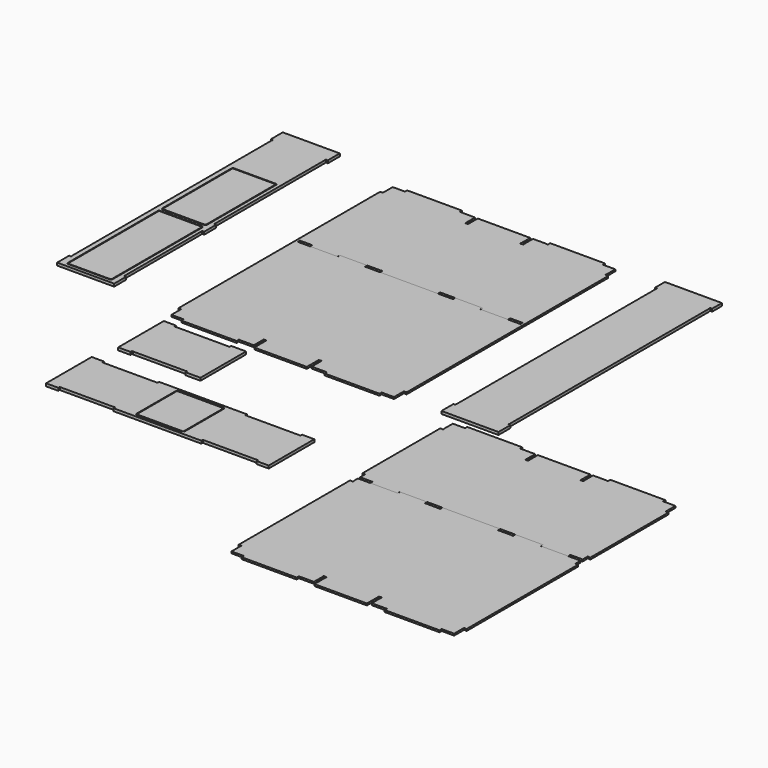
from build123d import *

# Parameters (mm, degrees)
F3_DEPTH  = 12
F5_DEPTH  = 18
F7_DEPTH  = 18
F9_DEPTH  = 18
F11_DEPTH = 12
F13_DEPTH = 12
F14_DEPTH = 18
F15_DEPTH = 12


with BuildPart() as f3:
    # F2 (on Top) → F3 (new body)
    with BuildSketch(Plane.XY):
        with BuildLine():
            Line((-993.5265209191, 1782.8284271247), (-1360.5265209191, 1782.8284271247))
            Line((-1360.5265209191, 1782.8284271247), (-1360.5265209191, 1770.8604506609))
            ThreePointArc((-1360.5265209191, 1770.8604506609), (-1359.5132677477, 1769.5012526055), (-1359.1540050798, 1767.8444388928))
            ThreePointArc((-1359.1540050798, 1767.8444388928), (-1359.5132677477, 1766.1876251801), (-1360.5265209191, 1764.8284271247))
            ThreePointArc((-1360.5265209191, 1764.8284271247), (-1363.1540050798, 1763.8444388928), (-1365.7814892405, 1764.8284271247))
            Line((-1365.7814892405, 1764.8284271247), (-1442.5265209191, 1764.8284271247))
            Line((-1442.5265209191, 1764.8284271247), (-1442.5265209191, 1688.4852813742))
            ThreePointArc((-1442.5265209191, 1688.4852813742), (-1441.6594299138, 1687.187587979), (-1441.3549480438, 1685.6568542495))
            ThreePointArc((-1441.3549480438, 1685.6568542495), (-1441.6594299138, 1684.12612052), (-1442.5265209191, 1682.8284271247))
            ThreePointArc((-1442.5265209191, 1682.8284271247), (-1445.3549480438, 1681.6568542495), (-1448.1833751686, 1682.8284271247))
            Line((-1448.1833751686, 1682.8284271247), (-1460.5265209191, 1682.8284271247))
            Line((-1460.5265209191, 1682.8284271247), (-1460.5265209191, 993.8284271247))
            Line((-1460.5265209191, 993.8284271247), (-1460.5265209191, 991.8284271247))
            Line((-1460.5265209191, 991.8284271247), (-1442.5265209191, 991.8284271247))
            Line((-1442.5265209191, 991.8284271247), (-1366.1833751686, 991.8284271247))
            ThreePointArc((-1366.1833751686, 991.8284271247), (-1363.3549480438, 993), (-1360.5265209191, 991.8284271247))
            ThreePointArc((-1360.5265209191, 991.8284271247), (-1359.6594299138, 990.5307337295), (-1359.3549480438, 989))
            ThreePointArc((-1359.3549480438, 989), (-1359.6594299138, 987.4692662705), (-1360.5265209191, 986.1715728753))
            Line((-1360.5265209191, 986.1715728753), (-1360.5265209191, 973.8284271247))
            Line((-1360.5265209191, 973.8284271247), (-1182.6833751686, 973.8284271247))
            Line((-1182.6833751686, 973.8284271247), (-1177.0265209191, 973.8284271247))
            Line((-1177.0265209191, 973.8284271247), (-1177.0265209191, 979.4852813742))
            Line((-1177.0265209191, 979.4852813742), (-1177.0265209191, 986.1715728753))
            ThreePointArc((-1177.0265209191, 986.1715728753), (-1178.1980937943, 989), (-1177.0265209191, 991.8284271247))
            ThreePointArc((-1177.0265209191, 991.8284271247), (-1174.1980937943, 993), (-1171.3696666696, 991.8284271247))
            Line((-1171.3696666696, 991.8284271247), (-993.5265209191, 991.8284271247))
            Line((-993.5265209191, 991.8284271247), (-899.1833751686, 991.8284271247))
            ThreePointArc((-899.1833751686, 991.8284271247), (-896.3549480438, 993), (-893.5265209191, 991.8284271247))
            ThreePointArc((-893.5265209191, 991.8284271247), (-892.6594299138, 990.5307337295), (-892.3549480438, 989))
            ThreePointArc((-892.3549480438, 989), (-892.6594299138, 987.4692662705), (-893.5265209191, 986.1715728753))
            Line((-893.5265209191, 986.1715728753), (-893.5265209191, 973.8284271247))
            Line((-893.5265209191, 973.8284271247), (-507.5265209191, 973.8284271247))
            Line((-507.5265209191, 973.8284271247), (-507.5265209191, 986.1715728753))
            ThreePointArc((-507.5265209191, 986.1715728753), (-508.6980937943, 989), (-507.5265209191, 991.8284271247))
            ThreePointArc((-507.5265209191, 991.8284271247), (-504.6980937943, 993), (-501.8696666696, 991.8284271247))
            Line((-501.8696666696, 991.8284271247), (-407.5265209191, 991.8284271247))
            Line((-407.5265209191, 991.8284271247), (-229.6833751686, 991.8284271247))
            ThreePointArc((-229.6833751686, 991.8284271247), (-226.8549480438, 993), (-224.0265209191, 991.8284271247))
            ThreePointArc((-224.0265209191, 991.8284271247), (-222.8549480438, 989), (-224.0265209191, 986.1715728753))
            Line((-224.0265209191, 986.1715728753), (-224.0265209191, 979.4852813742))
            Line((-224.0265209191, 979.4852813742), (-224.0265209191, 973.8284271247))
            Line((-224.0265209191, 973.8284271247), (-218.3696666696, 973.8284271247))
            Line((-218.3696666696, 973.8284271247), (-40.5265209191, 973.8284271247))
            Line((-40.5265209191, 973.8284271247), (-40.5265209191, 986.1715728753))
            ThreePointArc((-40.5265209191, 986.1715728753), (-41.6980937943, 989), (-40.5265209191, 991.8284271247))
            ThreePointArc((-40.5265209191, 991.8284271247), (-37.6980937943, 993), (-34.8696666696, 991.8284271247))
            Line((-34.8696666696, 991.8284271247), (41.4734790809, 991.8284271247))
            Line((41.4734790809, 991.8284271247), (59.4734790809, 991.8284271247))
            Line((59.4734790809, 991.8284271247), (59.4734790809, 993.8284271247))
            Line((59.4734790809, 993.8284271247), (59.4734790809, 1682.8284271247))
            Line((59.4734790809, 1682.8284271247), (47.1303333304, 1682.8284271247))
            ThreePointArc((47.1303333304, 1682.8284271247), (44.3019062057, 1681.6568542495), (41.4734790809, 1682.8284271247))
            ThreePointArc((41.4734790809, 1682.8284271247), (40.3019062057, 1685.6568542495), (41.4734790809, 1688.4852813742))
            Line((41.4734790809, 1688.4852813742), (41.4734790809, 1764.8284271247))
            Line((41.4734790809, 1764.8284271247), (-35.2715525977, 1764.8284271247))
            ThreePointArc((-35.2715525977, 1764.8284271247), (-37.8990367584, 1763.8444388928), (-40.5265209191, 1764.8284271247))
            ThreePointArc((-40.5265209191, 1764.8284271247), (-41.8990367584, 1767.8444388928), (-40.5265209191, 1770.8604506609))
            Line((-40.5265209191, 1770.8604506609), (-40.5265209191, 1782.8284271247))
            Line((-40.5265209191, 1782.8284271247), (-407.5265209191, 1782.8284271247))
            Line((-407.5265209191, 1782.8284271247), (-407.5265209191, 1770.4852813742))
            ThreePointArc((-407.5265209191, 1770.4852813742), (-406.6594299138, 1769.187587979), (-406.3549480438, 1767.6568542495))
            ThreePointArc((-406.3549480438, 1767.6568542495), (-406.6594299138, 1766.12612052), (-407.5265209191, 1764.8284271247))
            ThreePointArc((-407.5265209191, 1764.8284271247), (-410.3549480438, 1763.6568542495), (-413.1833751686, 1764.8284271247))
            Line((-413.1833751686, 1764.8284271247), (-507.5265209191, 1764.8284271247))
            Line((-507.5265209191, 1764.8284271247), (-507.5265209191, 1688.4852813742))
            ThreePointArc((-507.5265209191, 1688.4852813742), (-506.6594299138, 1687.187587979), (-506.3549480438, 1685.6568542495))
            ThreePointArc((-506.3549480438, 1685.6568542495), (-506.6594299138, 1684.12612052), (-507.5265209191, 1682.8284271247))
            ThreePointArc((-507.5265209191, 1682.8284271247), (-510.3549480438, 1681.6568542495), (-513.1833751686, 1682.8284271247))
            Line((-513.1833751686, 1682.8284271247), (-519.8696666696, 1682.8284271247))
            ThreePointArc((-519.8696666696, 1682.8284271247), (-522.6980937943, 1681.6568542495), (-525.5265209191, 1682.8284271247))
            ThreePointArc((-525.5265209191, 1682.8284271247), (-526.6980937943, 1685.6568542495), (-525.5265209191, 1688.4852813742))
            Line((-525.5265209191, 1688.4852813742), (-525.5265209191, 1764.8284271247))
            Line((-525.5265209191, 1764.8284271247), (-875.5265209191, 1764.8284271247))
            Line((-875.5265209191, 1764.8284271247), (-875.5265209191, 1688.4852813742))
            ThreePointArc((-875.5265209191, 1688.4852813742), (-874.6594299138, 1687.187587979), (-874.3549480438, 1685.6568542495))
            ThreePointArc((-874.3549480438, 1685.6568542495), (-874.6594299138, 1684.12612052), (-875.5265209191, 1682.8284271247))
            ThreePointArc((-875.5265209191, 1682.8284271247), (-878.3549480438, 1681.6568542495), (-881.1833751686, 1682.8284271247))
            Line((-881.1833751686, 1682.8284271247), (-887.8696666696, 1682.8284271247))
            ThreePointArc((-887.8696666696, 1682.8284271247), (-890.6980937943, 1681.6568542495), (-893.5265209191, 1682.8284271247))
            ThreePointArc((-893.5265209191, 1682.8284271247), (-894.6980937943, 1685.6568542495), (-893.5265209191, 1688.4852813742))
            Line((-893.5265209191, 1688.4852813742), (-893.5265209191, 1764.8284271247))
            Line((-893.5265209191, 1764.8284271247), (-987.8696666696, 1764.8284271247))
            ThreePointArc((-987.8696666696, 1764.8284271247), (-990.6980937943, 1763.6568542495), (-993.5265209191, 1764.8284271247))
            ThreePointArc((-993.5265209191, 1764.8284271247), (-994.6980937943, 1767.6568542495), (-993.5265209191, 1770.4852813742))
            Line((-993.5265209191, 1770.4852813742), (-993.5265209191, 1782.8284271247))
        make_face()
    extrude(amount=F3_DEPTH)


with BuildPart() as f5:
    # F4 (on Top) → F5 (new body)
    with BuildSketch(Plane.XY):
        with BuildLine():
            Line((719.4346694946, 1723.644810468), (719.4346694946, 1805.644810468))
            Line((719.4346694946, 1805.644810468), (339.4346694946, 1805.644810468))
            Line((339.4346694946, 1805.644810468), (339.4346694946, 1723.644810468))
            Line((339.4346694946, 1723.644810468), (346.7778152451, 1723.644810468))
            ThreePointArc((346.7778152451, 1723.644810468), (349.6062423699, 1724.8163833432), (352.4346694946, 1723.644810468))
            Line((352.4346694946, 1723.644810468), (707.4346694946, 1723.644810468))
            ThreePointArc((707.4346694946, 1723.644810468), (710.2630966194, 1724.8163833432), (713.0915237441, 1723.644810468))
            Line((713.0915237441, 1723.644810468), (719.4346694946, 1723.644810468))
        make_face()
        with BuildLine():
            Line((719.4346694946, -56.355189532), (719.4346694946, 43.644810468))
            Line((719.4346694946, 43.644810468), (713.0915237441, 43.644810468))
            ThreePointArc((713.0915237441, 43.644810468), (710.2630966194, 42.4732375927), (707.4346694946, 43.644810468))
            Line((707.4346694946, 43.644810468), (352.4346694946, 43.644810468))
            ThreePointArc((352.4346694946, 43.644810468), (349.6062423699, 42.4732375927), (346.7778152451, 43.644810468))
            Line((346.7778152451, 43.644810468), (339.4346694946, 43.644810468))
            Line((339.4346694946, 43.644810468), (339.4346694946, -56.355189532))
            Line((339.4346694946, -56.355189532), (719.4346694946, -56.355189532))
        make_face()
        with BuildLine():
            ThreePointArc((707.4346694946, 1717.9879562185), (706.2630966194, 1720.8163833432), (707.4346694946, 1723.644810468))
            Line((707.4346694946, 1723.644810468), (352.4346694946, 1723.644810468))
            ThreePointArc((352.4346694946, 1723.644810468), (353.3017604999, 1722.3471170727), (353.6062423699, 1720.8163833432))
            ThreePointArc((353.6062423699, 1720.8163833432), (353.3017604999, 1719.2856496138), (352.4346694946, 1717.9879562185))
            Line((352.4346694946, 1717.9879562185), (352.4346694946, 49.3016647175))
            ThreePointArc((352.4346694946, 49.3016647175), (353.3017604999, 48.0039713222), (353.6062423699, 46.4732375927))
            ThreePointArc((353.6062423699, 46.4732375927), (353.3017604999, 44.9425038632), (352.4346694946, 43.644810468))
            Line((352.4346694946, 43.644810468), (707.4346694946, 43.644810468))
            ThreePointArc((707.4346694946, 43.644810468), (706.2630966194, 46.4732375927), (707.4346694946, 49.3016647175))
            Line((707.4346694946, 49.3016647175), (707.4346694946, 1717.9879562185))
        make_face()
    extrude(amount=F5_DEPTH)


with BuildPart() as f7:
    # F6 (on Top) → F7 (new body)
    with BuildSketch(Plane.XY):
        with BuildLine():
            Line((-1340.3959202766, -167.9005670547), (-1422.3959202766, -167.9005670547))
            Line((-1422.3959202766, -167.9005670547), (-1422.3959202766, -180.9005670547))
            Line((-1422.3959202766, -180.9005670547), (-1422.3959202766, -547.9005670547))
            Line((-1422.3959202766, -547.9005670547), (-1340.3959202766, -547.9005670547))
            Line((-1340.3959202766, -547.9005670547), (-1340.3959202766, -541.5574213042))
            ThreePointArc((-1340.3959202766, -541.5574213042), (-1341.5674931519, -538.7289941795), (-1340.3959202766, -535.9005670547))
            ThreePointArc((-1340.3959202766, -535.9005670547), (-1337.5674931519, -534.7289941795), (-1334.7390660271, -535.9005670547))
            Line((-1334.7390660271, -535.9005670547), (-979.5527745261, -535.9005670547))
            ThreePointArc((-979.5527745261, -535.9005670547), (-976.7243474014, -534.7289941795), (-973.8959202766, -535.9005670547))
            ThreePointArc((-973.8959202766, -535.9005670547), (-973.0288292713, -537.19826045), (-972.7243474014, -538.7289941795))
            ThreePointArc((-972.7243474014, -538.7289941795), (-973.0288292713, -540.259727909), (-973.8959202766, -541.5574213042))
            Line((-973.8959202766, -541.5574213042), (-973.8959202766, -547.9005670547))
            Line((-973.8959202766, -547.9005670547), (-873.8959202766, -547.9005670547))
            Line((-873.8959202766, -547.9005670547), (-873.8959202766, -180.9005670547))
            Line((-873.8959202766, -180.9005670547), (-873.8959202766, -167.9005670547))
            Line((-873.8959202766, -167.9005670547), (-973.8959202766, -167.9005670547))
            Line((-973.8959202766, -167.9005670547), (-973.8959202766, -175.2437128053))
            ThreePointArc((-973.8959202766, -175.2437128053), (-973.0288292713, -176.5414062005), (-972.7243474014, -178.07213993))
            ThreePointArc((-972.7243474014, -178.07213993), (-973.0288292713, -179.6028736595), (-973.8959202766, -180.9005670547))
            ThreePointArc((-973.8959202766, -180.9005670547), (-976.7243474014, -182.07213993), (-979.5527745261, -180.9005670547))
            Line((-979.5527745261, -180.9005670547), (-1334.7390660271, -180.9005670547))
            ThreePointArc((-1334.7390660271, -180.9005670547), (-1337.5674931519, -182.07213993), (-1340.3959202766, -180.9005670547))
            ThreePointArc((-1340.3959202766, -180.9005670547), (-1341.5674931519, -178.07213993), (-1340.3959202766, -175.2437128053))
            Line((-1340.3959202766, -175.2437128053), (-1340.3959202766, -167.9005670547))
        make_face()
    extrude(amount=F7_DEPTH)


with BuildPart() as f9:
    # F8 (on Top) → F9 (new body)
    with BuildSketch(Plane.XY):
        with BuildLine():
            Line((-1900.4519424438, 1780), (-1900.4519424438, 1880))
            Line((-1900.4519424438, 1880), (-2267.4519424438, 1880))
            Line((-2267.4519424438, 1880), (-2267.4519424438, 1780))
            Line((-2267.4519424438, 1780), (-2261.1087966933, 1780))
            ThreePointArc((-2261.1087966933, 1780), (-2258.2803695686, 1781.1715728753), (-2255.4519424438, 1780))
            ThreePointArc((-2255.4519424438, 1780), (-2254.5848514385, 1778.7023066047), (-2254.2803695686, 1777.1715728753))
            ThreePointArc((-2254.2803695686, 1777.1715728753), (-2254.5848514385, 1775.6408391458), (-2255.4519424438, 1774.3431457505))
            Line((-2255.4519424438, 1774.3431457505), (-2255.4519424438, 105.6568542495))
            ThreePointArc((-2255.4519424438, 105.6568542495), (-2254.5848514385, 104.3591608542), (-2254.2803695686, 102.8284271247))
            ThreePointArc((-2254.2803695686, 102.8284271247), (-2254.5848514385, 101.2976933953), (-2255.4519424438, 100))
            ThreePointArc((-2255.4519424438, 100), (-2258.2803695686, 98.8284271247), (-2261.1087966933, 100))
            Line((-2261.1087966933, 100), (-2267.4519424438, 100))
            Line((-2267.4519424438, 100), (-2267.4519424438, 0))
            Line((-2267.4519424438, 0), (-1900.4519424438, 0))
            Line((-1900.4519424438, 0), (-1900.4519424438, 100))
            ThreePointArc((-1900.4519424438, 100), (-1901.6235153191, 102.8284271247), (-1900.4519424438, 105.6568542495))
            Line((-1900.4519424438, 105.6568542495), (-1900.4519424438, 744.3431457505))
            ThreePointArc((-1900.4519424438, 744.3431457505), (-1901.6235153191, 747.1715728753), (-1900.4519424438, 750))
            Line((-1900.4519424438, 750), (-1900.4519424438, 850))
            ThreePointArc((-1900.4519424438, 850), (-1901.6235153191, 852.8284271247), (-1900.4519424438, 855.6568542495))
            Line((-1900.4519424438, 855.6568542495), (-1900.4519424438, 1774.3431457505))
            ThreePointArc((-1900.4519424438, 1774.3431457505), (-1901.6235153191, 1777.1715728753), (-1900.4519424438, 1780))
        make_face()
        with BuildLine():
            ThreePointArc((-2222.4519424438, 781), (-2219.5230102557, 788.0710678119), (-2212.4519424438, 791))
            Line((-2212.4519424438, 791), (-1934.4519424438, 791))
            ThreePointArc((-1934.4519424438, 791), (-1927.380874632, 788.0710678119), (-1924.4519424438, 781))
            Line((-1924.4519424438, 781), (-1924.4519424438, 32))
            ThreePointArc((-1924.4519424438, 32), (-1927.380874632, 24.9289321881), (-1934.4519424438, 22))
            Line((-1934.4519424438, 22), (-2212.4519424438, 22))
            ThreePointArc((-2212.4519424438, 22), (-2219.5230102557, 24.9289321881), (-2222.4519424438, 32))
            Line((-2222.4519424438, 32), (-2222.4519424438, 781))
        make_face(mode=Mode.SUBTRACT)
        with BuildLine():
            ThreePointArc((-2222.4519424438, 1395), (-2219.5230102557, 1402.0710678119), (-2212.4519424438, 1405))
            Line((-2212.4519424438, 1405), (-1934.4519424438, 1405))
            ThreePointArc((-1934.4519424438, 1405), (-1927.380874632, 1402.0710678119), (-1924.4519424438, 1395))
            Line((-1924.4519424438, 1395), (-1924.4519424438, 819))
            ThreePointArc((-1924.4519424438, 819), (-1927.380874632, 811.9289321881), (-1934.4519424438, 809))
            Line((-1934.4519424438, 809), (-2212.4519424438, 809))
            ThreePointArc((-2212.4519424438, 809), (-2219.5230102557, 811.9289321881), (-2222.4519424438, 819))
            Line((-2222.4519424438, 819), (-2222.4519424438, 1395))
        make_face(mode=Mode.SUBTRACT)
        with BuildLine():
            Line((-1887.4519424438, 1780), (-1887.4519424438, 1880))
            Line((-1887.4519424438, 1880), (-1900.4519424438, 1880))
            Line((-1900.4519424438, 1880), (-1900.4519424438, 1780))
            ThreePointArc((-1900.4519424438, 1780), (-1897.6235153191, 1781.1715728753), (-1894.7950881944, 1780))
            Line((-1894.7950881944, 1780), (-1887.4519424438, 1780))
        make_face()
        with BuildLine():
            Line((-1887.4519424438, 750), (-1887.4519424438, 850))
            Line((-1887.4519424438, 850), (-1894.7950881944, 850))
            ThreePointArc((-1894.7950881944, 850), (-1897.6235153191, 848.8284271247), (-1900.4519424438, 850))
            Line((-1900.4519424438, 850), (-1900.4519424438, 750))
            ThreePointArc((-1900.4519424438, 750), (-1897.6235153191, 751.1715728753), (-1894.7950881944, 750))
            Line((-1894.7950881944, 750), (-1887.4519424438, 750))
        make_face()
        with BuildLine():
            Line((-1887.4519424438, 0), (-1887.4519424438, 100))
            Line((-1887.4519424438, 100), (-1894.7950881944, 100))
            ThreePointArc((-1894.7950881944, 100), (-1897.6235153191, 98.8284271247), (-1900.4519424438, 100))
            Line((-1900.4519424438, 100), (-1900.4519424438, 0))
            Line((-1900.4519424438, 0), (-1887.4519424438, 0))
        make_face()
    extrude(amount=F9_DEPTH)


with BuildPart() as f9b:
    # F8 (on Top) → F9, piece 2 (new body)
    with BuildSketch(Plane.XY):
        with BuildLine():
            Line((-1934.4519424438, 1400), (-2212.4519424438, 1400))
            ThreePointArc((-2212.4519424438, 1400), (-2215.9874763498, 1398.5355339059), (-2217.4519424438, 1395))
            Line((-2217.4519424438, 1395), (-2217.4519424438, 819))
            ThreePointArc((-2217.4519424438, 819), (-2215.9874763498, 815.4644660941), (-2212.4519424438, 814))
            Line((-2212.4519424438, 814), (-1934.4519424438, 814))
            ThreePointArc((-1934.4519424438, 814), (-1930.9164085379, 815.4644660941), (-1929.4519424438, 819))
            Line((-1929.4519424438, 819), (-1929.4519424438, 1395))
            ThreePointArc((-1929.4519424438, 1395), (-1930.9164085379, 1398.5355339059), (-1934.4519424438, 1400))
        make_face()
    extrude(amount=F9_DEPTH)


with BuildPart() as f9c:
    # F8 (on Top) → F9, piece 3 (new body)
    with BuildSketch(Plane.XY):
        with BuildLine():
            ThreePointArc((-2217.4519424438, 32), (-2215.9874763498, 28.4644660941), (-2212.4519424438, 27))
            Line((-2212.4519424438, 27), (-1934.4519424438, 27))
            ThreePointArc((-1934.4519424438, 27), (-1930.9164085379, 28.4644660941), (-1929.4519424438, 32))
            Line((-1929.4519424438, 32), (-1929.4519424438, 781))
            ThreePointArc((-1929.4519424438, 781), (-1930.9164085379, 784.5355339059), (-1934.4519424438, 786))
            Line((-1934.4519424438, 786), (-2212.4519424438, 786))
            ThreePointArc((-2212.4519424438, 786), (-2215.9874763498, 784.5355339059), (-2217.4519424438, 781))
            Line((-2217.4519424438, 781), (-2217.4519424438, 32))
        make_face()
    extrude(amount=F9_DEPTH)


with BuildPart() as f11:
    # F10 (on Top) → F11 (new body)
    with BuildSketch(Plane.XY):
        with BuildLine():
            Line((916.9637542371, -104.4519302007), (549.9637542371, -104.4519302007))
            Line((549.9637542371, -104.4519302007), (549.9637542371, -116.7950759512))
            ThreePointArc((549.9637542371, -116.7950759512), (550.8308452424, -118.0927693465), (551.1353271124, -119.623503076))
            ThreePointArc((551.1353271124, -119.623503076), (550.8308452424, -121.1542368054), (549.9637542371, -122.4519302007))
            ThreePointArc((549.9637542371, -122.4519302007), (547.1353271124, -123.623503076), (544.3068999876, -122.4519302007))
            Line((544.3068999876, -122.4519302007), (467.9637542371, -122.4519302007))
            Line((467.9637542371, -122.4519302007), (467.9637542371, -198.7950759512))
            ThreePointArc((467.9637542371, -198.7950759512), (468.8308452424, -200.0927693465), (469.1353271124, -201.623503076))
            ThreePointArc((469.1353271124, -201.623503076), (468.8308452424, -203.1542368054), (467.9637542371, -204.4519302007))
            ThreePointArc((467.9637542371, -204.4519302007), (465.1353271124, -205.623503076), (462.3068999876, -204.4519302007))
            Line((462.3068999876, -204.4519302007), (449.9637542371, -204.4519302007))
            Line((449.9637542371, -204.4519302007), (449.9637542371, -853.4519302007))
            Line((449.9637542371, -853.4519302007), (462.3068999876, -853.4519302007))
            ThreePointArc((462.3068999876, -853.4519302007), (465.1353271124, -852.2803573255), (467.9637542371, -853.4519302007))
            ThreePointArc((467.9637542371, -853.4519302007), (468.8308452424, -854.749623596), (469.1353271124, -856.2803573255))
            ThreePointArc((469.1353271124, -856.2803573255), (468.8308452424, -857.8110910549), (467.9637542371, -859.1087844502))
            Line((467.9637542371, -859.1087844502), (467.9637542371, -895.4519302008))
            Line((467.9637542371, -895.4519302008), (543.5485567773, -895.4519302008))
            ThreePointArc((543.5485567773, -895.4519302008), (546.7561555072, -893.8417650043), (549.9637542371, -895.4519302008))
            ThreePointArc((549.9637542371, -895.4519302008), (550.5528906125, -896.5828755968), (550.7561555072, -897.8417650043))
            ThreePointArc((550.7561555072, -897.8417650043), (550.5528906125, -899.1006544117), (549.9637542371, -900.2315998078))
            Line((549.9637542371, -900.2315998078), (549.9637542371, -913.4519302007))
            Line((549.9637542371, -913.4519302007), (727.8068999876, -913.4519302007))
            Line((727.8068999876, -913.4519302007), (733.4637542371, -913.4519302007))
            Line((733.4637542371, -913.4519302007), (733.4637542371, -907.7950759512))
            Line((733.4637542371, -907.7950759512), (733.4637542371, -901.1087844502))
            ThreePointArc((733.4637542371, -901.1087844502), (732.2921813618, -898.2803573255), (733.4637542371, -895.4519302007))
            ThreePointArc((733.4637542371, -895.4519302007), (736.2921813618, -894.2803573255), (739.1206084866, -895.4519302007))
            Line((739.1206084866, -895.4519302007), (916.9637542371, -895.4519302007))
            Line((916.9637542371, -895.4519302007), (1016.9637542371, -895.4519302007))
            Line((1016.9637542371, -895.4519302007), (1402.9637542371, -895.4519302007))
            Line((1402.9637542371, -895.4519302007), (1502.9637542371, -895.4519302007))
            Line((1502.9637542371, -895.4519302007), (1680.8068999876, -895.4519302007))
            ThreePointArc((1680.8068999876, -895.4519302007), (1683.6353271124, -894.2803573255), (1686.4637542371, -895.4519302007))
            ThreePointArc((1686.4637542371, -895.4519302007), (1687.6353271124, -898.2803573255), (1686.4637542371, -901.1087844502))
            Line((1686.4637542371, -901.1087844502), (1686.4637542371, -907.7950759512))
            Line((1686.4637542371, -907.7950759512), (1686.4637542371, -913.4519302007))
            Line((1686.4637542371, -913.4519302007), (1692.1206084866, -913.4519302007))
            Line((1692.1206084866, -913.4519302007), (1869.9637542371, -913.4519302007))
            Line((1869.9637542371, -913.4519302007), (1869.9637542371, -900.2315998078))
            ThreePointArc((1869.9637542371, -900.2315998078), (1869.171352967, -897.8417650043), (1869.9637542371, -895.4519302007))
            ThreePointArc((1869.9637542371, -895.4519302007), (1873.171352967, -893.8417650043), (1876.3789516969, -895.4519302007))
            Line((1876.3789516969, -895.4519302007), (1951.9637542371, -895.4519302007))
            Line((1951.9637542371, -895.4519302007), (1951.9637542371, -859.1087844502))
            ThreePointArc((1951.9637542371, -859.1087844502), (1950.7921813618, -856.2803573255), (1951.9637542371, -853.4519302007))
            ThreePointArc((1951.9637542371, -853.4519302007), (1954.7921813618, -852.2803573255), (1957.6206084866, -853.4519302007))
            Line((1957.6206084866, -853.4519302007), (1969.9637542371, -853.4519302007))
            Line((1969.9637542371, -853.4519302007), (1969.9637542371, -204.4519302007))
            Line((1969.9637542371, -204.4519302007), (1957.6206084866, -204.4519302007))
            ThreePointArc((1957.6206084866, -204.4519302007), (1954.7921813618, -205.623503076), (1951.9637542371, -204.4519302007))
            ThreePointArc((1951.9637542371, -204.4519302007), (1950.7921813618, -201.623503076), (1951.9637542371, -198.7950759512))
            Line((1951.9637542371, -198.7950759512), (1951.9637542371, -122.4519302007))
            Line((1951.9637542371, -122.4519302007), (1875.6206084866, -122.4519302007))
            ThreePointArc((1875.6206084866, -122.4519302007), (1872.7921813618, -123.623503076), (1869.9637542371, -122.4519302007))
            ThreePointArc((1869.9637542371, -122.4519302007), (1868.7921813618, -119.623503076), (1869.9637542371, -116.7950759512))
            Line((1869.9637542371, -116.7950759512), (1869.9637542371, -104.4519302007))
            Line((1869.9637542371, -104.4519302007), (1502.9637542371, -104.4519302007))
            Line((1502.9637542371, -104.4519302007), (1502.9637542371, -116.7950759512))
            ThreePointArc((1502.9637542371, -116.7950759512), (1503.8308452424, -118.0927693465), (1504.1353271124, -119.623503076))
            ThreePointArc((1504.1353271124, -119.623503076), (1503.8308452424, -121.1542368054), (1502.9637542371, -122.4519302007))
            ThreePointArc((1502.9637542371, -122.4519302007), (1500.1353271124, -123.623503076), (1497.3068999876, -122.4519302007))
            Line((1497.3068999876, -122.4519302007), (1402.9637542371, -122.4519302007))
            Line((1402.9637542371, -122.4519302007), (1402.9637542371, -198.7950759512))
            ThreePointArc((1402.9637542371, -198.7950759512), (1403.8308452424, -200.0927693465), (1404.1353271124, -201.623503076))
            ThreePointArc((1404.1353271124, -201.623503076), (1403.8308452424, -203.1542368054), (1402.9637542371, -204.4519302007))
            ThreePointArc((1402.9637542371, -204.4519302007), (1400.1353271124, -205.623503076), (1397.3068999876, -204.4519302007))
            Line((1397.3068999876, -204.4519302007), (1390.6206084866, -204.4519302007))
            ThreePointArc((1390.6206084866, -204.4519302007), (1387.7921813618, -205.623503076), (1384.9637542371, -204.4519302007))
            ThreePointArc((1384.9637542371, -204.4519302007), (1383.7921813618, -201.623503076), (1384.9637542371, -198.7950759512))
            Line((1384.9637542371, -198.7950759512), (1384.9637542371, -122.4519302007))
            Line((1384.9637542371, -122.4519302007), (1034.9637542371, -122.4519302007))
            Line((1034.9637542371, -122.4519302007), (1034.9637542371, -198.7950759512))
            ThreePointArc((1034.9637542371, -198.7950759512), (1035.8308452424, -200.0927693465), (1036.1353271124, -201.623503076))
            ThreePointArc((1036.1353271124, -201.623503076), (1035.8308452424, -203.1542368054), (1034.9637542371, -204.4519302007))
            ThreePointArc((1034.9637542371, -204.4519302007), (1032.1353271124, -205.623503076), (1029.3068999876, -204.4519302007))
            Line((1029.3068999876, -204.4519302007), (1022.6206084866, -204.4519302007))
            ThreePointArc((1022.6206084866, -204.4519302007), (1019.7921813618, -205.623503076), (1016.9637542371, -204.4519302007))
            ThreePointArc((1016.9637542371, -204.4519302007), (1015.7921813618, -201.623503076), (1016.9637542371, -198.7950759512))
            Line((1016.9637542371, -198.7950759512), (1016.9637542371, -122.4519302007))
            Line((1016.9637542371, -122.4519302007), (922.6206084866, -122.4519302007))
            ThreePointArc((922.6206084866, -122.4519302007), (919.7921813618, -123.623503076), (916.9637542371, -122.4519302007))
            ThreePointArc((916.9637542371, -122.4519302007), (915.7921813618, -119.623503076), (916.9637542371, -116.7950759512))
            Line((916.9637542371, -116.7950759512), (916.9637542371, -104.4519302007))
        make_face()
    extrude(amount=F11_DEPTH)


with BuildPart() as f13:
    # F2 (on Top) → F13 (new body)
    with BuildSketch(Plane.XY):
        with BuildLine():
            Line((-1442.5265209191, 991.8284271247), (-1460.5265209191, 991.8284271247))
            Line((-1460.5265209191, 991.8284271247), (-1460.5265209191, 973.8284271247))
            Line((-1460.5265209191, 973.8284271247), (-1460.5265209191, 2.8284271247))
            Line((-1460.5265209191, 2.8284271247), (-1448.1833751686, 2.8284271247))
            ThreePointArc((-1448.1833751686, 2.8284271247), (-1445.3549480438, 4), (-1442.5265209191, 2.8284271247))
            ThreePointArc((-1442.5265209191, 2.8284271247), (-1441.6594299138, 1.5307337295), (-1441.3549480438, 0))
            ThreePointArc((-1441.3549480438, 0), (-1441.6594299138, -1.5307337295), (-1442.5265209191, -2.8284271247))
            Line((-1442.5265209191, -2.8284271247), (-1442.5265209191, -79.1715728753))
            Line((-1442.5265209191, -79.1715728753), (-1366.1833751686, -79.1715728753))
            ThreePointArc((-1366.1833751686, -79.1715728753), (-1363.3549480438, -78), (-1360.5265209191, -79.1715728753))
            ThreePointArc((-1360.5265209191, -79.1715728753), (-1359.6594299138, -80.4692662705), (-1359.3549480438, -82))
            ThreePointArc((-1359.3549480438, -82), (-1359.6594299138, -83.5307337295), (-1360.5265209191, -84.8284271247))
            Line((-1360.5265209191, -84.8284271247), (-1360.5265209191, -97.1715728753))
            Line((-1360.5265209191, -97.1715728753), (-993.5265209191, -97.1715728753))
            Line((-993.5265209191, -97.1715728753), (-993.5265209191, -84.8284271247))
            ThreePointArc((-993.5265209191, -84.8284271247), (-994.6980937943, -82), (-993.5265209191, -79.1715728753))
            ThreePointArc((-993.5265209191, -79.1715728753), (-990.6980937943, -78), (-987.8696666696, -79.1715728753))
            Line((-987.8696666696, -79.1715728753), (-893.5265209191, -79.1715728753))
            Line((-893.5265209191, -79.1715728753), (-893.5265209191, -2.8284271247))
            ThreePointArc((-893.5265209191, -2.8284271247), (-894.6980937943, 0), (-893.5265209191, 2.8284271247))
            ThreePointArc((-893.5265209191, 2.8284271247), (-890.6980937943, 4), (-887.8696666696, 2.8284271247))
            Line((-887.8696666696, 2.8284271247), (-881.1833751686, 2.8284271247))
            ThreePointArc((-881.1833751686, 2.8284271247), (-878.3549480438, 4), (-875.5265209191, 2.8284271247))
            ThreePointArc((-875.5265209191, 2.8284271247), (-874.6594299138, 1.5307337295), (-874.3549480438, 0))
            ThreePointArc((-874.3549480438, 0), (-874.6594299138, -1.5307337295), (-875.5265209191, -2.8284271247))
            Line((-875.5265209191, -2.8284271247), (-875.5265209191, -97.1715728753))
            Line((-875.5265209191, -97.1715728753), (-525.5265209191, -97.1715728753))
            Line((-525.5265209191, -97.1715728753), (-525.5265209191, -2.8284271247))
            ThreePointArc((-525.5265209191, -2.8284271247), (-526.6980937943, 0), (-525.5265209191, 2.8284271247))
            ThreePointArc((-525.5265209191, 2.8284271247), (-522.6980937943, 4), (-519.8696666696, 2.8284271247))
            Line((-519.8696666696, 2.8284271247), (-513.1833751686, 2.8284271247))
            ThreePointArc((-513.1833751686, 2.8284271247), (-510.3549480438, 4), (-507.5265209191, 2.8284271247))
            ThreePointArc((-507.5265209191, 2.8284271247), (-506.6594299138, 1.5307337295), (-506.3549480438, 0))
            ThreePointArc((-506.3549480438, 0), (-506.6594299138, -1.5307337295), (-507.5265209191, -2.8284271247))
            Line((-507.5265209191, -2.8284271247), (-507.5265209191, -79.1715728753))
            Line((-507.5265209191, -79.1715728753), (-413.1833751686, -79.1715728753))
            ThreePointArc((-413.1833751686, -79.1715728753), (-410.3549480438, -78), (-407.5265209191, -79.1715728753))
            ThreePointArc((-407.5265209191, -79.1715728753), (-406.6594299138, -80.4692662705), (-406.3549480438, -82))
            ThreePointArc((-406.3549480438, -82), (-406.6594299138, -83.5307337295), (-407.5265209191, -84.8284271247))
            Line((-407.5265209191, -84.8284271247), (-407.5265209191, -97.1715728753))
            Line((-407.5265209191, -97.1715728753), (-40.5265209191, -97.1715728753))
            Line((-40.5265209191, -97.1715728753), (-40.5265209191, -84.8284271247))
            ThreePointArc((-40.5265209191, -84.8284271247), (-41.6980937943, -82), (-40.5265209191, -79.1715728753))
            ThreePointArc((-40.5265209191, -79.1715728753), (-37.6980937943, -78), (-34.8696666696, -79.1715728753))
            Line((-34.8696666696, -79.1715728753), (41.4734790809, -79.1715728753))
            Line((41.4734790809, -79.1715728753), (41.4734790809, -2.8284271247))
            ThreePointArc((41.4734790809, -2.8284271247), (40.3019062057, 0), (41.4734790809, 2.8284271247))
            ThreePointArc((41.4734790809, 2.8284271247), (44.3019062057, 4), (47.1303333304, 2.8284271247))
            Line((47.1303333304, 2.8284271247), (59.4734790809, 2.8284271247))
            Line((59.4734790809, 2.8284271247), (59.4734790809, 991.8284271247))
            Line((59.4734790809, 991.8284271247), (41.4734790809, 991.8284271247))
            Line((41.4734790809, 991.8284271247), (41.4734790809, 979.4852813742))
            ThreePointArc((41.4734790809, 979.4852813742), (42.3405700862, 978.187587979), (42.6450519562, 976.6568542495))
            ThreePointArc((42.6450519562, 976.6568542495), (42.3405700862, 975.12612052), (41.4734790809, 973.8284271247))
            ThreePointArc((41.4734790809, 973.8284271247), (38.6450519562, 972.6568542495), (35.8166248314, 973.8284271247))
            Line((35.8166248314, 973.8284271247), (-40.5265209191, 973.8284271247))
            Line((-40.5265209191, 973.8284271247), (-218.3696666696, 973.8284271247))
            ThreePointArc((-218.3696666696, 973.8284271247), (-221.1980937943, 972.6568542495), (-224.0265209191, 973.8284271247))
            ThreePointArc((-224.0265209191, 973.8284271247), (-225.1980937943, 976.6568542495), (-224.0265209191, 979.4852813742))
            Line((-224.0265209191, 979.4852813742), (-224.0265209191, 986.1715728753))
            Line((-224.0265209191, 986.1715728753), (-224.0265209191, 991.8284271247))
            Line((-224.0265209191, 991.8284271247), (-229.6833751686, 991.8284271247))
            Line((-229.6833751686, 991.8284271247), (-407.5265209191, 991.8284271247))
            Line((-407.5265209191, 991.8284271247), (-407.5265209191, 979.4852813742))
            ThreePointArc((-407.5265209191, 979.4852813742), (-406.6594299138, 978.187587979), (-406.3549480438, 976.6568542495))
            ThreePointArc((-406.3549480438, 976.6568542495), (-406.6594299138, 975.12612052), (-407.5265209191, 973.8284271247))
            ThreePointArc((-407.5265209191, 973.8284271247), (-410.3549480438, 972.6568542495), (-413.1833751686, 973.8284271247))
            Line((-413.1833751686, 973.8284271247), (-507.5265209191, 973.8284271247))
            Line((-507.5265209191, 973.8284271247), (-893.5265209191, 973.8284271247))
            Line((-893.5265209191, 973.8284271247), (-987.8696666696, 973.8284271247))
            ThreePointArc((-987.8696666696, 973.8284271247), (-990.6980937943, 972.6568542495), (-993.5265209191, 973.8284271247))
            ThreePointArc((-993.5265209191, 973.8284271247), (-994.6980937943, 976.6568542495), (-993.5265209191, 979.4852813742))
            Line((-993.5265209191, 979.4852813742), (-993.5265209191, 991.8284271247))
            Line((-993.5265209191, 991.8284271247), (-1171.3696666696, 991.8284271247))
            Line((-1171.3696666696, 991.8284271247), (-1177.0265209191, 991.8284271247))
            Line((-1177.0265209191, 991.8284271247), (-1177.0265209191, 986.1715728753))
            Line((-1177.0265209191, 986.1715728753), (-1177.0265209191, 979.4852813742))
            ThreePointArc((-1177.0265209191, 979.4852813742), (-1175.8549480438, 976.6568542495), (-1177.0265209191, 973.8284271247))
            ThreePointArc((-1177.0265209191, 973.8284271247), (-1179.8549480438, 972.6568542495), (-1182.6833751686, 973.8284271247))
            Line((-1182.6833751686, 973.8284271247), (-1360.5265209191, 973.8284271247))
            Line((-1360.5265209191, 973.8284271247), (-1436.8696666696, 973.8284271247))
            ThreePointArc((-1436.8696666696, 973.8284271247), (-1439.6980937943, 972.6568542495), (-1442.5265209191, 973.8284271247))
            ThreePointArc((-1442.5265209191, 973.8284271247), (-1443.6980937943, 976.6568542495), (-1442.5265209191, 979.4852813742))
            Line((-1442.5265209191, 979.4852813742), (-1442.5265209191, 991.8284271247))
        make_face()
    extrude(amount=F13_DEPTH)


with BuildPart() as f14:
    # F12 (on Top) → F14 (new body)
    with BuildSketch(Plane.XY):
        with BuildLine():
            Line((-1402, -691.7245292664), (-1484, -691.7245292664))
            Line((-1484, -691.7245292664), (-1484, -704.7245292664))
            Line((-1484, -704.7245292664), (-1484, -1059.7245292664))
            Line((-1484, -1059.7245292664), (-1484, -1071.7245292664))
            Line((-1484, -1071.7245292664), (-1402, -1071.7245292664))
            Line((-1402, -1071.7245292664), (-1402, -1065.3813835158))
            ThreePointArc((-1402, -1065.3813835158), (-1403.1715728753, -1062.5529563911), (-1402, -1059.7245292664))
            ThreePointArc((-1402, -1059.7245292664), (-1399.1715728753, -1058.5529563911), (-1396.3431457505, -1059.7245292664))
            Line((-1396.3431457505, -1059.7245292664), (-1040.6568542495, -1059.7245292664))
            ThreePointArc((-1040.6568542495, -1059.7245292664), (-1037.8284271247, -1058.5529563911), (-1035, -1059.7245292664))
            ThreePointArc((-1035, -1059.7245292664), (-1034.1329089947, -1061.0222226616), (-1033.8284271247, -1062.5529563911))
            ThreePointArc((-1033.8284271247, -1062.5529563911), (-1034.1329089947, -1064.0836901206), (-1035, -1065.3813835158))
            Line((-1035, -1065.3813835158), (-1035, -1071.7245292664))
            Line((-1035, -1071.7245292664), (-925.3927507401, -1071.7245292664))
            Line((-925.3927507401, -1071.7245292664), (-449, -1071.7245292664))
            Line((-449, -1071.7245292664), (-449, -1065.3813835158))
            ThreePointArc((-449, -1065.3813835158), (-450.1715728753, -1062.5529563911), (-449, -1059.7245292664))
            ThreePointArc((-449, -1059.7245292664), (-446.1715728753, -1058.5529563911), (-443.3431457505, -1059.7245292664))
            Line((-443.3431457505, -1059.7245292664), (-87.6568542495, -1059.7245292664))
            ThreePointArc((-87.6568542495, -1059.7245292664), (-84.8284271247, -1058.5529563911), (-82, -1059.7245292664))
            ThreePointArc((-82, -1059.7245292664), (-81.1329089947, -1061.0222226616), (-80.8284271247, -1062.5529563911))
            ThreePointArc((-80.8284271247, -1062.5529563911), (-81.1329089947, -1064.0836901206), (-82, -1065.3813835158))
            Line((-82, -1065.3813835158), (-82, -1071.7245292664))
            Line((-82, -1071.7245292664), (0, -1071.7245292664))
            Line((0, -1071.7245292664), (0, -691.7245292664))
            Line((0, -691.7245292664), (-82, -691.7245292664))
            Line((-82, -691.7245292664), (-82, -699.0676750169))
            ThreePointArc((-82, -699.0676750169), (-81.1329089947, -700.3653684122), (-80.8284271247, -701.8961021416))
            ThreePointArc((-80.8284271247, -701.8961021416), (-81.1329089947, -703.4268358711), (-82, -704.7245292664))
            ThreePointArc((-82, -704.7245292664), (-84.8284271247, -705.8961021416), (-87.6568542495, -704.7245292664))
            Line((-87.6568542495, -704.7245292664), (-443.3431457505, -704.7245292664))
            ThreePointArc((-443.3431457505, -704.7245292664), (-446.1715728753, -705.8961021416), (-449, -704.7245292664))
            ThreePointArc((-449, -704.7245292664), (-450.1715728753, -701.8961021416), (-449, -699.0676750169))
            Line((-449, -699.0676750169), (-449, -691.7245292664))
            Line((-449, -691.7245292664), (-1035, -691.7245292664))
            Line((-1035, -691.7245292664), (-1035, -699.0676750169))
            ThreePointArc((-1035, -699.0676750169), (-1034.1329089947, -700.3653684122), (-1033.8284271247, -701.8961021416))
            ThreePointArc((-1033.8284271247, -701.8961021416), (-1034.1329089947, -703.4268358711), (-1035, -704.7245292664))
            ThreePointArc((-1035, -704.7245292664), (-1037.8284271247, -705.8961021416), (-1040.6568542495, -704.7245292664))
            Line((-1040.6568542495, -704.7245292664), (-1396.3431457505, -704.7245292664))
            ThreePointArc((-1396.3431457505, -704.7245292664), (-1399.1715728753, -705.8961021416), (-1402, -704.7245292664))
            ThreePointArc((-1402, -704.7245292664), (-1403.1715728753, -701.8961021416), (-1402, -699.0676750169))
            Line((-1402, -699.0676750169), (-1402, -691.7245292664))
        make_face()
        with BuildLine():
            Line((-892.3927507401, -708.7245292664), (-742, -708.7245292664))
            Line((-742, -708.7245292664), (-591.6072492599, -708.7245292664))
            ThreePointArc((-591.6072492599, -708.7245292664), (-584.5361814481, -711.6534614545), (-581.6072492599, -718.7245292664))
            Line((-581.6072492599, -718.7245292664), (-581.6072492599, -1044.7245292664))
            ThreePointArc((-581.6072492599, -1044.7245292664), (-584.5361814481, -1051.7955970782), (-591.6072492599, -1054.7245292664))
            Line((-591.6072492599, -1054.7245292664), (-742, -1054.7245292664))
            Line((-742, -1054.7245292664), (-892.3927507401, -1054.7245292664))
            ThreePointArc((-892.3927507401, -1054.7245292664), (-899.4638185519, -1051.7955970782), (-902.3927507401, -1044.7245292664))
            Line((-902.3927507401, -1044.7245292664), (-902.3927507401, -718.7245292664))
            ThreePointArc((-902.3927507401, -718.7245292664), (-899.4638185519, -711.6534614545), (-892.3927507401, -708.7245292664))
        make_face(mode=Mode.SUBTRACT)
    extrude(amount=-F14_DEPTH)


with BuildPart() as f14b:
    # F12 (on Top) → F14, piece 2 (new body)
    with BuildSketch(Plane.XY):
        with BuildLine():
            Line((-892.3927507401, -1049.7245292664), (-732.3927507401, -1049.7245292664))
            Line((-732.3927507401, -1049.7245292664), (-591.6072492599, -1049.7245292664))
            ThreePointArc((-591.6072492599, -1049.7245292664), (-588.071715354, -1048.2600631723), (-586.6072492599, -1044.7245292664))
            Line((-586.6072492599, -1044.7245292664), (-586.6072492599, -718.7245292664))
            ThreePointArc((-586.6072492599, -718.7245292664), (-588.071715354, -715.1889953604), (-591.6072492599, -713.7245292664))
            Line((-591.6072492599, -713.7245292664), (-732.3927507401, -713.7245292664))
            Line((-732.3927507401, -713.7245292664), (-892.3927507401, -713.7245292664))
            ThreePointArc((-892.3927507401, -713.7245292664), (-895.928284646, -715.1889953604), (-897.3927507401, -718.7245292664))
            Line((-897.3927507401, -718.7245292664), (-897.3927507401, -1044.7245292664))
            ThreePointArc((-897.3927507401, -1044.7245292664), (-895.928284646, -1048.2600631723), (-892.3927507401, -1049.7245292664))
        make_face()
    extrude(amount=-F14_DEPTH)


with BuildPart() as f15:
    # F10 (on Top) → F15 (new body)
    with BuildSketch(Plane.XY):
        with BuildLine():
            Line((462.3068999876, -955.4519302007), (449.9637542371, -955.4519302007))
            Line((449.9637542371, -955.4519302007), (449.9637542371, -1884.4519302007))
            Line((449.9637542371, -1884.4519302007), (462.3068999876, -1884.4519302007))
            ThreePointArc((462.3068999876, -1884.4519302007), (465.1353271124, -1883.2803573255), (467.9637542371, -1884.4519302007))
            ThreePointArc((467.9637542371, -1884.4519302007), (468.8308452424, -1885.749623596), (469.1353271124, -1887.2803573255))
            ThreePointArc((469.1353271124, -1887.2803573255), (468.8308452424, -1888.8110910549), (467.9637542371, -1890.1087844502))
            Line((467.9637542371, -1890.1087844502), (467.9637542371, -1966.4519302007))
            Line((467.9637542371, -1966.4519302007), (544.3068999876, -1966.4519302007))
            ThreePointArc((544.3068999876, -1966.4519302007), (547.1353271124, -1965.2803573255), (549.9637542371, -1966.4519302007))
            ThreePointArc((549.9637542371, -1966.4519302007), (550.8308452424, -1967.749623596), (551.1353271124, -1969.2803573255))
            ThreePointArc((551.1353271124, -1969.2803573255), (550.8308452424, -1970.8110910549), (549.9637542371, -1972.1087844502))
            Line((549.9637542371, -1972.1087844502), (549.9637542371, -1984.4519302007))
            Line((549.9637542371, -1984.4519302007), (916.9637542371, -1984.4519302007))
            Line((916.9637542371, -1984.4519302007), (916.9637542371, -1972.1087844502))
            ThreePointArc((916.9637542371, -1972.1087844502), (915.7921813618, -1969.2803573255), (916.9637542371, -1966.4519302007))
            ThreePointArc((916.9637542371, -1966.4519302007), (919.7921813618, -1965.2803573255), (922.6206084866, -1966.4519302007))
            Line((922.6206084866, -1966.4519302007), (1016.9637542371, -1966.4519302007))
            Line((1016.9637542371, -1966.4519302007), (1016.9637542371, -1890.1087844502))
            ThreePointArc((1016.9637542371, -1890.1087844502), (1015.7921813618, -1887.2803573255), (1016.9637542371, -1884.4519302007))
            ThreePointArc((1016.9637542371, -1884.4519302007), (1019.7921813618, -1883.2803573255), (1022.6206084866, -1884.4519302007))
            Line((1022.6206084866, -1884.4519302007), (1029.3068999876, -1884.4519302007))
            ThreePointArc((1029.3068999876, -1884.4519302007), (1032.1353271124, -1883.2803573255), (1034.9637542371, -1884.4519302007))
            ThreePointArc((1034.9637542371, -1884.4519302007), (1035.8308452424, -1885.749623596), (1036.1353271124, -1887.2803573255))
            ThreePointArc((1036.1353271124, -1887.2803573255), (1035.8308452424, -1888.8110910549), (1034.9637542371, -1890.1087844502))
            Line((1034.9637542371, -1890.1087844502), (1034.9637542371, -1984.4519302007))
            Line((1034.9637542371, -1984.4519302007), (1384.9637542371, -1984.4519302007))
            Line((1384.9637542371, -1984.4519302007), (1384.9637542371, -1890.1087844502))
            ThreePointArc((1384.9637542371, -1890.1087844502), (1383.7921813618, -1887.2803573255), (1384.9637542371, -1884.4519302007))
            ThreePointArc((1384.9637542371, -1884.4519302007), (1387.7921813618, -1883.2803573255), (1390.6206084866, -1884.4519302007))
            Line((1390.6206084866, -1884.4519302007), (1397.3068999876, -1884.4519302007))
            ThreePointArc((1397.3068999876, -1884.4519302007), (1400.1353271124, -1883.2803573255), (1402.9637542371, -1884.4519302007))
            ThreePointArc((1402.9637542371, -1884.4519302007), (1403.8308452424, -1885.749623596), (1404.1353271124, -1887.2803573255))
            ThreePointArc((1404.1353271124, -1887.2803573255), (1403.8308452424, -1888.8110910549), (1402.9637542371, -1890.1087844502))
            Line((1402.9637542371, -1890.1087844502), (1402.9637542371, -1966.4519302007))
            Line((1402.9637542371, -1966.4519302007), (1497.3068999876, -1966.4519302007))
            ThreePointArc((1497.3068999876, -1966.4519302007), (1500.1353271124, -1965.2803573255), (1502.9637542371, -1966.4519302007))
            ThreePointArc((1502.9637542371, -1966.4519302007), (1503.8308452424, -1967.749623596), (1504.1353271124, -1969.2803573255))
            ThreePointArc((1504.1353271124, -1969.2803573255), (1503.8308452424, -1970.8110910549), (1502.9637542371, -1972.1087844502))
            Line((1502.9637542371, -1972.1087844502), (1502.9637542371, -1984.4519302007))
            Line((1502.9637542371, -1984.4519302007), (1869.9637542371, -1984.4519302007))
            Line((1869.9637542371, -1984.4519302007), (1869.9637542371, -1972.1087844502))
            ThreePointArc((1869.9637542371, -1972.1087844502), (1868.7921813618, -1969.2803573255), (1869.9637542371, -1966.4519302007))
            ThreePointArc((1869.9637542371, -1966.4519302007), (1872.7921813618, -1965.2803573255), (1875.6206084866, -1966.4519302007))
            Line((1875.6206084866, -1966.4519302007), (1951.9637542371, -1966.4519302007))
            Line((1951.9637542371, -1966.4519302007), (1951.9637542371, -1890.1087844502))
            ThreePointArc((1951.9637542371, -1890.1087844502), (1950.7921813618, -1887.2803573255), (1951.9637542371, -1884.4519302007))
            ThreePointArc((1951.9637542371, -1884.4519302007), (1954.7921813618, -1883.2803573255), (1957.6206084866, -1884.4519302007))
            Line((1957.6206084866, -1884.4519302007), (1969.9637542371, -1884.4519302007))
            Line((1969.9637542371, -1884.4519302007), (1969.9637542371, -955.4519302007))
            Line((1969.9637542371, -955.4519302007), (1957.6206084866, -955.4519302007))
            ThreePointArc((1957.6206084866, -955.4519302007), (1954.7921813618, -956.623503076), (1951.9637542371, -955.4519302007))
            ThreePointArc((1951.9637542371, -955.4519302007), (1950.7921813618, -952.623503076), (1951.9637542371, -949.7950759512))
            Line((1951.9637542371, -949.7950759512), (1951.9637542371, -913.4519302007))
            Line((1951.9637542371, -913.4519302007), (1869.9637542371, -913.4519302007))
            Line((1869.9637542371, -913.4519302007), (1692.1206084866, -913.4519302007))
            ThreePointArc((1692.1206084866, -913.4519302007), (1689.2921813618, -914.623503076), (1686.4637542371, -913.4519302007))
            ThreePointArc((1686.4637542371, -913.4519302007), (1685.2921813618, -910.623503076), (1686.4637542371, -907.7950759512))
            Line((1686.4637542371, -907.7950759512), (1686.4637542371, -901.1087844502))
            Line((1686.4637542371, -901.1087844502), (1686.4637542371, -895.4519302007))
            Line((1686.4637542371, -895.4519302007), (1680.8068999876, -895.4519302007))
            Line((1680.8068999876, -895.4519302007), (1502.9637542371, -895.4519302007))
            Line((1502.9637542371, -895.4519302007), (1502.9637542371, -907.7950759512))
            ThreePointArc((1502.9637542371, -907.7950759512), (1503.8308452424, -909.0927693465), (1504.1353271124, -910.623503076))
            ThreePointArc((1504.1353271124, -910.623503076), (1503.8308452424, -912.1542368054), (1502.9637542371, -913.4519302007))
            ThreePointArc((1502.9637542371, -913.4519302007), (1500.1353271124, -914.623503076), (1497.3068999876, -913.4519302007))
            Line((1497.3068999876, -913.4519302007), (1408.6206084866, -913.4519302007))
            ThreePointArc((1408.6206084866, -913.4519302007), (1405.7921813618, -914.623503076), (1402.9637542371, -913.4519302007))
            ThreePointArc((1402.9637542371, -913.4519302007), (1401.7921813618, -910.623503076), (1402.9637542371, -907.7950759512))
            Line((1402.9637542371, -907.7950759512), (1402.9637542371, -895.4519302007))
            Line((1402.9637542371, -895.4519302007), (1016.9637542371, -895.4519302007))
            Line((1016.9637542371, -895.4519302007), (1016.9637542371, -907.7950759512))
            ThreePointArc((1016.9637542371, -907.7950759512), (1017.8308452424, -909.0927693465), (1018.1353271124, -910.623503076))
            ThreePointArc((1018.1353271124, -910.623503076), (1017.8308452424, -912.1542368054), (1016.9637542371, -913.4519302007))
            ThreePointArc((1016.9637542371, -913.4519302007), (1014.1353271124, -914.623503076), (1011.3068999876, -913.4519302007))
            Line((1011.3068999876, -913.4519302007), (922.6206084866, -913.4519302007))
            ThreePointArc((922.6206084866, -913.4519302007), (919.7921813618, -914.623503076), (916.9637542371, -913.4519302007))
            ThreePointArc((916.9637542371, -913.4519302007), (915.7921813618, -910.623503076), (916.9637542371, -907.7950759512))
            Line((916.9637542371, -907.7950759512), (916.9637542371, -895.4519302007))
            Line((916.9637542371, -895.4519302007), (739.1206084866, -895.4519302007))
            Line((739.1206084866, -895.4519302007), (733.4637542371, -895.4519302007))
            Line((733.4637542371, -895.4519302007), (733.4637542371, -901.1087844502))
            Line((733.4637542371, -901.1087844502), (733.4637542371, -907.7950759512))
            ThreePointArc((733.4637542371, -907.7950759512), (734.6353271124, -910.623503076), (733.4637542371, -913.4519302007))
            ThreePointArc((733.4637542371, -913.4519302007), (730.6353271124, -914.623503076), (727.8068999876, -913.4519302007))
            Line((727.8068999876, -913.4519302007), (549.9637542371, -913.4519302007))
            Line((549.9637542371, -913.4519302007), (467.9637542371, -913.4519302007))
            Line((467.9637542371, -913.4519302007), (467.9637542371, -949.7950759512))
            ThreePointArc((467.9637542371, -949.7950759512), (468.8308452424, -951.0927693465), (469.1353271124, -952.623503076))
            ThreePointArc((469.1353271124, -952.623503076), (468.8308452424, -954.1542368054), (467.9637542371, -955.4519302007))
            ThreePointArc((467.9637542371, -955.4519302007), (465.1353271124, -956.623503076), (462.3068999876, -955.4519302007))
        make_face()
    extrude(amount=F15_DEPTH)


solid = Compound([f3.part, f5.part, f7.part, f9.part, f9b.part, f9c.part, f11.part, f13.part, f14.part, f14b.part, f15.part])
